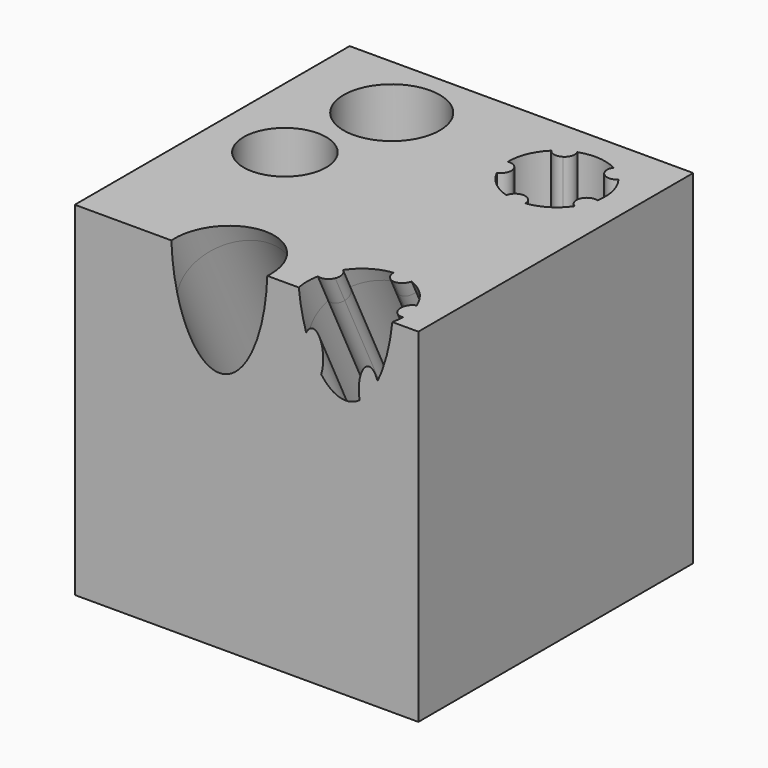
from build123d import *

# Parameters (mm, degrees)
F0_W           = 15
F0_H           = 15
F1_DEPTH       = 15
F2_R           = 2.1
F3_DEPTH       = 10
F4_DEPTH       = 10
F6_D           = 3.6
F6_DEPTH       = 10
F6_TIP         = 1.0815491142
F9_R           = 2.1
F10_DEPTH      = 10
F10_DEPTH_BACK = 10
F11_DEPTH      = 10
F11_DEPTH_BACK = 10


with BuildPart() as f1:
    # F0 (on Top) → F1 (new body)
    with BuildSketch(Plane.XY):
        Rectangle(F0_W, F0_H)
    extrude(amount=F1_DEPTH)

    # F2 (on face) → F3 (cut)
    with BuildSketch(Plane.XY.offset(15)):
        with Locations((-3.3081052825, 4.5566549525)):
            Circle(F2_R)
    extrude(amount=-F3_DEPTH, mode=Mode.SUBTRACT)

    # F2 (on face) → F4 (cut)
    with BuildSketch(Plane.XY.offset(15)):
        with BuildLine():
            ThreePointArc((3.2809909909, 5.6586071096), (4.271900841, 5.899439318), (5.2151213678, 5.5118344659))
            ThreePointArc((5.2151213678, 5.5118344659), (5.0605091693, 5.7942622045), (5.1341789855, 6.1076997863))
            ThreePointArc((5.1341789855, 6.1076997863), (4.3059514618, 6.3481491967), (3.450923876, 6.2354346119))
            ThreePointArc((3.450923876, 6.2354346119), (3.4764516514, 5.9144693594), (3.2809909909, 5.6586071096))
        make_face()
        with BuildLine():
            ThreePointArc((3.5456670252, 2.2421209971), (3.7136732609, 2.5167921893), (4.0221963108, 2.608900206))
            ThreePointArc((4.0221963108, 2.608900206), (3.0789758, 2.9965050415), (2.5437227765, 3.8644950423))
            ThreePointArc((2.5437227765, 3.8644950423), (2.5027997945, 3.5451274527), (2.2589656824, 3.334853171))
            ThreePointArc((2.2589656824, 3.334853171), (2.787683207, 2.6535055877), (3.5456670252, 2.2421209971))
        make_face()
        with BuildLine():
            ThreePointArc((5.8747835443, 3.0604646595), (5.6654725032, 3.3051261397), (5.6732114262, 3.6270119283))
            ThreePointArc((5.6732114262, 3.6270119283), (5.0131061422, 2.8497324056), (4.0221963108, 2.608900206))
            ThreePointArc((4.0221963108, 2.608900206), (4.313287058, 2.471290132), (4.4379209082, 2.174411775))
            ThreePointArc((4.4379209082, 2.174411775), (5.2493036675, 2.4667040397), (5.8747835443, 3.0604646595))
        make_face()
        with BuildLine():
            ThreePointArc((5.2151213678, 5.5118344659), (5.644516455, 4.9470549944), (5.7970485739, 4.2541697621))
            ThreePointArc((5.7970485739, 4.2541697621), (5.7657932583, 3.9345361486), (5.6732114262, 3.6270119283))
            ThreePointArc((5.6732114262, 3.6270119283), (5.8940383698, 3.8613318458), (6.2149004544, 3.8881252289))
            ThreePointArc((6.2149004544, 3.8881252289), (6.1876450529, 4.7501193664), (5.816229058, 5.5284682012))
            ThreePointArc((5.816229058, 5.5284682012), (5.5188614887, 5.4050061266), (5.2151213678, 5.5118344659))
        make_face()
        with BuildLine():
            ThreePointArc((2.5437227765, 3.8644950423), (2.6208857067, 4.8813275594), (3.2809909909, 5.6586071096))
            ThreePointArc((3.2809909909, 5.6586071096), (2.9646084595, 5.598837153), (2.6892768391, 5.7657588495))
            ThreePointArc((2.6892768391, 5.7657588495), (2.2046594805, 5.0523706202), (2.0476393662, 4.204360341))
            ThreePointArc((2.0476393662, 4.204360341), (2.360783986, 4.1294549747), (2.5437227765, 3.8644950423))
        make_face()
        with BuildLine():
            ThreePointArc((5.6732114262, 3.6270119283), (5.7657932583, 3.9345361486), (5.7970485739, 4.2541697621))
            ThreePointArc((5.7970485739, 4.2541697621), (5.644516455, 4.9470549944), (5.2151213678, 5.5118344659))
            ThreePointArc((5.2151213678, 5.5118344659), (4.271900841, 5.899439318), (3.2809909909, 5.6586071096))
            ThreePointArc((3.2809909909, 5.6586071096), (2.6208857067, 4.8813275594), (2.5437227765, 3.8644950423))
            ThreePointArc((2.5437227765, 3.8644950423), (3.0789758, 2.9965050415), (4.0221963108, 2.608900206))
            ThreePointArc((4.0221963108, 2.608900206), (5.0131061422, 2.8497324056), (5.6732114262, 3.6270119283))
        make_face()
    extrude(amount=-F4_DEPTH, mode=Mode.SUBTRACT)

    # F6
    with Locations(Plane.XY.offset(15)):
        with Locations((-4.327217117, 0)):
            Hole(F6_D / 2, depth=F6_DEPTH)
            with Locations((0, 0, -(F6_DEPTH + F6_TIP / 2))):  # 118° drill point
                Cone(0, F6_D / 2, F6_TIP, mode=Mode.SUBTRACT)

    # F9 (on line) → F10 (cut, two sides)
    with BuildSketch(Plane(origin=(0, -6.5801176454, 13.4912404864), x_dir=(1, 0, 0), z_dir=(0, -0.4383711468, 0.8987940463))) as f10_sk:
        with Locations((-1.1891657487, 0)):
            Circle(F9_R)
    extrude(amount=-F10_DEPTH, mode=Mode.SUBTRACT)
    extrude(f10_sk.sketch, amount=F10_DEPTH_BACK, mode=Mode.SUBTRACT)

    # F9 (on line) → F11 (cut, two sides)
    with BuildSketch(Plane(origin=(0, -6.5801176454, 13.4912404864), x_dir=(1, 0, 0), z_dir=(0, -0.4383711468, 0.8987940463))) as f11_sk:
        with BuildLine():
            ThreePointArc((4.9336170518, -1.6870876514), (4.9217202173, -1.3653287012), (5.1278529304, -1.117983474))
            ThreePointArc((5.1278529304, -1.117983474), (4.1276234932, -1.3165874448), (3.2016843949, -0.8893413207))
            ThreePointArc((3.2016843949, -0.8893413207), (3.3441834561, -1.178070216), (3.2572910424, -1.4881025786))
            ThreePointArc((3.2572910424, -1.4881025786), (4.0745795038, -1.7634502148), (4.9336170518, -1.6870876514))
        make_face()
        with BuildLine():
            ThreePointArc((2.6004119701, -0.8804748841), (2.9027465931, -0.7697313384), (3.2016843949, -0.8893413207))
            ThreePointArc((3.2016843949, -0.8893413207), (2.7037129005, 0.0005613942), (2.823917186, 1.0132081149))
            ThreePointArc((2.823917186, 1.0132081149), (2.5933543197, 0.7884613294), (2.2716447953, 0.7752956598))
            ThreePointArc((2.2716447953, 0.7752956598), (2.2623296555, -0.0870789562), (2.6004119701, -0.8804748841))
        make_face()
        with BuildLine():
            ThreePointArc((5.1278529304, -1.117983474), (5.7454877945, -0.5126676326), (5.9721181259, 0.3219093778))
            ThreePointArc((5.9721181259, 0.3219093778), (5.9642004358, 0.483358092), (5.9405233533, 0.6432573507))
            ThreePointArc((5.9405233533, 0.6432573507), (5.4425518562, 1.5331600768), (4.5166127528, 1.9604062012))
            ThreePointArc((4.5166127528, 1.9604062012), (3.5163833114, 1.7618022241), (2.823917186, 1.0132081149))
            ThreePointArc((2.823917186, 1.0132081149), (2.7037129005, 0.0005613942), (3.2016843949, -0.8893413207))
            ThreePointArc((3.2016843949, -0.8893413207), (4.1276234932, -1.3165874448), (5.1278529304, -1.117983474))
        make_face()
        with BuildLine():
            ThreePointArc((5.9405233533, 0.6432573507), (5.9642004358, 0.483358092), (5.9721181259, 0.3219093778))
            ThreePointArc((5.9721181259, 0.3219093778), (5.7454877945, -0.5126676326), (5.1278529304, -1.117983474))
            ThreePointArc((5.1278529304, -1.117983474), (5.4464850598, -1.0716809479), (5.7144921267, -1.2501258132))
            ThreePointArc((5.7144921267, -1.2501258132), (6.2289193143, -0.5579253952), (6.4217514019, 0.2826651924))
            ThreePointArc((6.4217514019, 0.2826651924), (6.1120641324, 0.3707796135), (5.9405233533, 0.6432573507))
        make_face()
        with BuildLine():
            ThreePointArc((4.5166127528, 1.9604062012), (5.4425518562, 1.5331600768), (5.9405233533, 0.6432573507))
            ThreePointArc((5.9405233533, 0.6432573507), (5.9949497762, 0.9606027823), (6.2474796669, 1.1603501546))
            ThreePointArc((6.2474796669, 1.1603501546), (5.7481246921, 1.8635011762), (5.0082639284, 2.3066521666))
            ThreePointArc((5.0082639284, 2.3066521666), (4.8287635013, 2.039350922), (4.5166127528, 1.9604062012))
        make_face()
        with BuildLine():
            ThreePointArc((2.823917186, 1.0132081149), (3.5163833114, 1.7618022241), (4.5166127528, 1.9604062012))
            ThreePointArc((4.5166127528, 1.9604062012), (4.2316180075, 2.1102339389), (4.119682998, 2.4121294665))
            ThreePointArc((4.119682998, 2.4121294665), (3.2966374636, 2.1545002791), (2.646546277, 1.5877920657))
            ThreePointArc((2.646546277, 1.5877920657), (2.8452961865, 1.3344763829), (2.823917186, 1.0132081149))
        make_face()
    extrude(amount=-F11_DEPTH, mode=Mode.SUBTRACT)
    extrude(f11_sk.sketch, amount=F11_DEPTH_BACK, mode=Mode.SUBTRACT)


solid = f1.part
